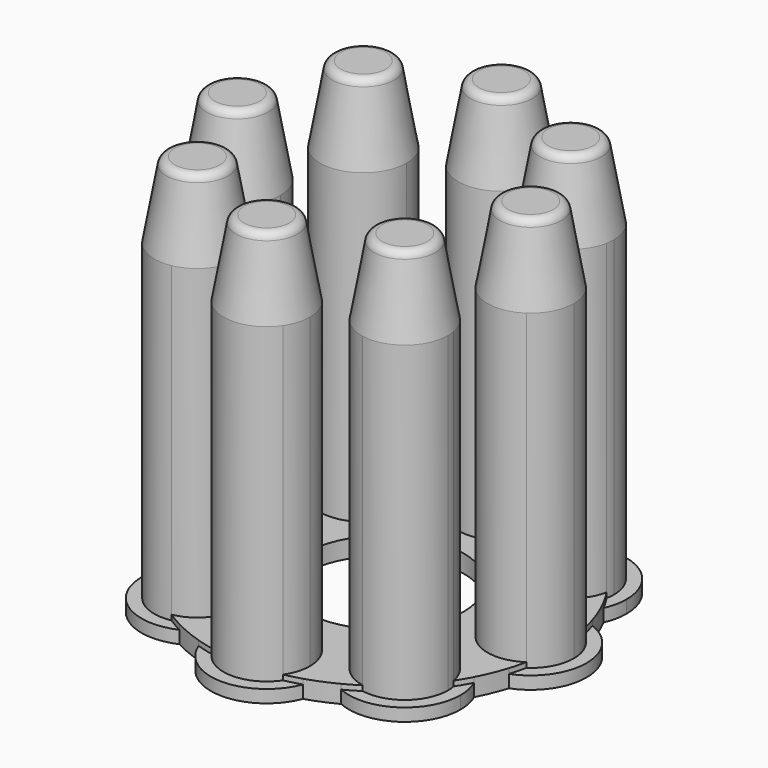
from build123d import *

# Parameters (mm, degrees)
F0_R            = 7.9375
F1_DEPTH        = 0.508
F2_DEPTH        = 1.27
F3_DEPTH        = 31.242
F5_COPIES_COUNT = 8


# Not quite as in the source:
# - a pattern or mirror of a feature is missing from the dataset's text; its kind, count and spacing are read off the source's solid


with BuildPart() as f1:
    # F0 (on Top) → F1 (new body)
    with BuildSketch(Plane.XY):
        with BuildLine():
            ThreePointArc((-5.219470135, 16.6642142857), (-1.0147277679, 9.1734047727), (5.588, 14.6685))
            ThreePointArc((5.588, 14.6685), (5.4950952273, 15.6832277679), (5.219470135, 16.6642142857))
            ThreePointArc((5.219470135, 16.6642142857), (4.4014869197, 16.8986928236), (3.573052384, 17.0930454545))
            ThreePointArc((3.573052384, 17.0930454545), (4.1275636999, 15.936704204), (4.318, 14.6685))
            ThreePointArc((4.318, 14.6685), (-1.268204204, 10.5409363001), (-3.573052384, 17.0930454545))
            ThreePointArc((-3.573052384, 17.0930454545), (-4.4014869197, 16.8986928236), (-5.219470135, 16.6642142857))
        make_face()
        with BuildLine():
            ThreePointArc((9.5600787818, 14.6131379223), (8.8368590405, 15.061501537), (8.0926561979, 15.4741016512))
            ThreePointArc((8.0926561979, 15.4741016512), (6.4208831266, 6.4208831266), (15.4741016512, 8.0926561979))
            ThreePointArc((15.4741016512, 8.0926561979), (15.061501537, 8.8368590405), (14.6131379223, 9.5600787818))
            ThreePointArc((14.6131379223, 9.5600787818), (7.3189087387, 7.3189087387), (9.5600787818, 14.6131379223))
        make_face()
        with BuildLine():
            ThreePointArc((17.0930454545, 3.573052384), (16.8986928236, 4.4014869197), (16.6642142857, 5.219470135))
            ThreePointArc((16.6642142857, 5.219470135), (9.0805, 0), (16.6642142857, -5.219470135))
            ThreePointArc((16.6642142857, -5.219470135), (16.8986928236, -4.4014869197), (17.0930454545, -3.573052384))
            ThreePointArc((17.0930454545, -3.573052384), (10.3505, 0), (17.0930454545, 3.573052384))
        make_face()
        with BuildLine():
            ThreePointArc((14.6131379223, -9.5600787818), (15.061501537, -8.8368590405), (15.4741016512, -8.0926561979))
            ThreePointArc((15.4741016512, -8.0926561979), (6.4208831266, -6.4208831266), (8.0926561979, -15.4741016512))
            ThreePointArc((8.0926561979, -15.4741016512), (8.8368590405, -15.061501537), (9.5600787818, -14.6131379223))
            ThreePointArc((9.5600787818, -14.6131379223), (7.3189087387, -7.3189087387), (14.6131379223, -9.5600787818))
        make_face()
        with BuildLine():
            ThreePointArc((3.573052384, -17.0930454545), (4.4014869197, -16.8986928236), (5.219470135, -16.6642142857))
            ThreePointArc((5.219470135, -16.6642142857), (5.4950952273, -15.6832277679), (5.588, -14.6685))
            ThreePointArc((5.588, -14.6685), (-1.0147277679, -9.1734047727), (-5.219470135, -16.6642142857))
            ThreePointArc((-5.219470135, -16.6642142857), (-4.4014869197, -16.8986928236), (-3.573052384, -17.0930454545))
            ThreePointArc((-3.573052384, -17.0930454545), (-1.268204204, -10.5409363001), (4.318, -14.6685))
            ThreePointArc((4.318, -14.6685), (4.1275636999, -15.936704204), (3.573052384, -17.0930454545))
        make_face()
        with BuildLine():
            ThreePointArc((-4.7841958198, -10.3721958198), (-9.2068001329, -4.907070305), (-15.4741016512, -8.0926561979))
            ThreePointArc((-15.4741016512, -8.0926561979), (-15.061501537, -8.8368590405), (-14.6131379223, -9.5600787818))
            ThreePointArc((-14.6131379223, -9.5600787818), (-9.9643134829, -6.0735034606), (-6.0541958198, -10.3721958198))
            ThreePointArc((-6.0541958198, -10.3721958198), (-7.044144936, -13.1234139709), (-9.5600787818, -14.6131379223))
            ThreePointArc((-9.5600787818, -14.6131379223), (-8.8368590405, -15.061501537), (-8.0926561979, -15.4741016512))
            ThreePointArc((-8.0926561979, -15.4741016512), (-5.6837093153, -13.4125639384), (-4.7841958198, -10.3721958198))
        make_face()
        with BuildLine():
            ThreePointArc((-9.0805, 0), (-11.5004017872, 4.6031399842), (-16.6642142857, 5.219470135))
            ThreePointArc((-16.6642142857, 5.219470135), (-16.8986928236, 4.4014869197), (-17.0930454545, 3.573052384))
            ThreePointArc((-17.0930454545, 3.573052384), (-12.6466275105, 3.8153840746), (-10.3505, 0))
            ThreePointArc((-10.3505, 0), (-12.6466275105, -3.8153840746), (-17.0930454545, -3.573052384))
            ThreePointArc((-17.0930454545, -3.573052384), (-16.8986928236, -4.4014869197), (-16.6642142857, -5.219470135))
            ThreePointArc((-16.6642142857, -5.219470135), (-11.5004017872, -4.6031399842), (-9.0805, 0))
        make_face()
        with BuildLine():
            ThreePointArc((-4.7841958198, 10.3721958198), (-5.6837093153, 13.4125639384), (-8.0926561979, 15.4741016512))
            ThreePointArc((-8.0926561979, 15.4741016512), (-8.8368590405, 15.061501537), (-9.5600787818, 14.6131379223))
            ThreePointArc((-9.5600787818, 14.6131379223), (-7.044144936, 13.1234139709), (-6.0541958198, 10.3721958198))
            ThreePointArc((-6.0541958198, 10.3721958198), (-9.9643134829, 6.0735034606), (-14.6131379223, 9.5600787818))
            ThreePointArc((-14.6131379223, 9.5600787818), (-15.061501537, 8.8368590405), (-15.4741016512, 8.0926561979))
            ThreePointArc((-15.4741016512, 8.0926561979), (-9.2068001329, 4.907070305), (-4.7841958198, 10.3721958198))
        make_face()
        with BuildLine():
            ThreePointArc((5.219470135, 16.6642142857), (5.4950952273, 15.6832277679), (5.588, 14.6685))
            ThreePointArc((5.588, 14.6685), (-1.0147277679, 9.1734047727), (-5.219470135, 16.6642142857))
            ThreePointArc((-5.219470135, 16.6642142857), (-6.6826094377, 16.1332463365), (-8.0926561979, 15.4741016512))
            ThreePointArc((-8.0926561979, 15.4741016512), (-5.6837093153, 13.4125639384), (-4.7841958198, 10.3721958198))
            ThreePointArc((-4.7841958198, 10.3721958198), (-9.2068001329, 4.907070305), (-15.4741016512, 8.0926561979))
            ThreePointArc((-15.4741016512, 8.0926561979), (-16.1332463365, 6.6826094377), (-16.6642142857, 5.219470135))
            ThreePointArc((-16.6642142857, 5.219470135), (-11.5004017872, 4.6031399842), (-9.0805, 0))
            ThreePointArc((-9.0805, 0), (-11.5004017872, -4.6031399842), (-16.6642142857, -5.219470135))
            ThreePointArc((-16.6642142857, -5.219470135), (-16.1332463365, -6.6826094377), (-15.4741016512, -8.0926561979))
            ThreePointArc((-15.4741016512, -8.0926561979), (-9.2068001329, -4.907070305), (-4.7841958198, -10.3721958198))
            ThreePointArc((-4.7841958198, -10.3721958198), (-5.6837093153, -13.4125639384), (-8.0926561979, -15.4741016512))
            ThreePointArc((-8.0926561979, -15.4741016512), (-6.6826094377, -16.1332463365), (-5.219470135, -16.6642142857))
            ThreePointArc((-5.219470135, -16.6642142857), (-1.0147277679, -9.1734047727), (5.588, -14.6685))
            ThreePointArc((5.588, -14.6685), (5.4950952273, -15.6832277679), (5.219470135, -16.6642142857))
            ThreePointArc((5.219470135, -16.6642142857), (6.6826094377, -16.1332463365), (8.0926561979, -15.4741016512))
            ThreePointArc((8.0926561979, -15.4741016512), (6.4208831266, -6.4208831266), (15.4741016512, -8.0926561979))
            ThreePointArc((15.4741016512, -8.0926561979), (16.1332463365, -6.6826094377), (16.6642142857, -5.219470135))
            ThreePointArc((16.6642142857, -5.219470135), (9.0805, 0), (16.6642142857, 5.219470135))
            ThreePointArc((16.6642142857, 5.219470135), (16.1332463365, 6.6826094377), (15.4741016512, 8.0926561979))
            ThreePointArc((15.4741016512, 8.0926561979), (6.4208831266, 6.4208831266), (8.0926561979, 15.4741016512))
            ThreePointArc((8.0926561979, 15.4741016512), (6.6826094377, 16.1332463365), (5.219470135, 16.6642142857))
        make_face()
        Circle(F0_R, mode=Mode.SUBTRACT)
    extrude(amount=F1_DEPTH)

    # F0 (on Top) → F2 (join)
    with BuildSketch(Plane.XY):
        with BuildLine():
            ThreePointArc((-5.219470135, 16.6642142857), (-1.0147277679, 9.1734047727), (5.588, 14.6685))
            ThreePointArc((5.588, 14.6685), (5.4950952273, 15.6832277679), (5.219470135, 16.6642142857))
            ThreePointArc((5.219470135, 16.6642142857), (4.4014869197, 16.8986928236), (3.573052384, 17.0930454545))
            ThreePointArc((3.573052384, 17.0930454545), (4.1275636999, 15.936704204), (4.318, 14.6685))
            ThreePointArc((4.318, 14.6685), (-1.268204204, 10.5409363001), (-3.573052384, 17.0930454545))
            ThreePointArc((-3.573052384, 17.0930454545), (-4.4014869197, 16.8986928236), (-5.219470135, 16.6642142857))
        make_face()
        with BuildLine():
            ThreePointArc((5.219470135, 16.6642142857), (5.4950952273, 15.6832277679), (5.588, 14.6685))
            ThreePointArc((5.588, 14.6685), (-1.0147277679, 9.1734047727), (-5.219470135, 16.6642142857))
            ThreePointArc((-5.219470135, 16.6642142857), (-6.6826094377, 16.1332463365), (-8.0926561979, 15.4741016512))
            ThreePointArc((-8.0926561979, 15.4741016512), (-5.6837093153, 13.4125639384), (-4.7841958198, 10.3721958198))
            ThreePointArc((-4.7841958198, 10.3721958198), (-9.2068001329, 4.907070305), (-15.4741016512, 8.0926561979))
            ThreePointArc((-15.4741016512, 8.0926561979), (-16.1332463365, 6.6826094377), (-16.6642142857, 5.219470135))
            ThreePointArc((-16.6642142857, 5.219470135), (-11.5004017872, 4.6031399842), (-9.0805, 0))
            ThreePointArc((-9.0805, 0), (-11.5004017872, -4.6031399842), (-16.6642142857, -5.219470135))
            ThreePointArc((-16.6642142857, -5.219470135), (-16.1332463365, -6.6826094377), (-15.4741016512, -8.0926561979))
            ThreePointArc((-15.4741016512, -8.0926561979), (-9.2068001329, -4.907070305), (-4.7841958198, -10.3721958198))
            ThreePointArc((-4.7841958198, -10.3721958198), (-5.6837093153, -13.4125639384), (-8.0926561979, -15.4741016512))
            ThreePointArc((-8.0926561979, -15.4741016512), (-6.6826094377, -16.1332463365), (-5.219470135, -16.6642142857))
            ThreePointArc((-5.219470135, -16.6642142857), (-1.0147277679, -9.1734047727), (5.588, -14.6685))
            ThreePointArc((5.588, -14.6685), (5.4950952273, -15.6832277679), (5.219470135, -16.6642142857))
            ThreePointArc((5.219470135, -16.6642142857), (6.6826094377, -16.1332463365), (8.0926561979, -15.4741016512))
            ThreePointArc((8.0926561979, -15.4741016512), (6.4208831266, -6.4208831266), (15.4741016512, -8.0926561979))
            ThreePointArc((15.4741016512, -8.0926561979), (16.1332463365, -6.6826094377), (16.6642142857, -5.219470135))
            ThreePointArc((16.6642142857, -5.219470135), (9.0805, 0), (16.6642142857, 5.219470135))
            ThreePointArc((16.6642142857, 5.219470135), (16.1332463365, 6.6826094377), (15.4741016512, 8.0926561979))
            ThreePointArc((15.4741016512, 8.0926561979), (6.4208831266, 6.4208831266), (8.0926561979, 15.4741016512))
            ThreePointArc((8.0926561979, 15.4741016512), (6.6826094377, 16.1332463365), (5.219470135, 16.6642142857))
        make_face()
        Circle(F0_R, mode=Mode.SUBTRACT)
        with BuildLine():
            ThreePointArc((3.573052384, 17.0930454545), (4.4014869197, 16.8986928236), (5.219470135, 16.6642142857))
            ThreePointArc((5.219470135, 16.6642142857), (0, 20.2565), (-5.219470135, 16.6642142857))
            ThreePointArc((-5.219470135, 16.6642142857), (-4.4014869197, 16.8986928236), (-3.573052384, 17.0930454545))
            ThreePointArc((-3.573052384, 17.0930454545), (0, 18.9865), (3.573052384, 17.0930454545))
        make_face()
        with BuildLine():
            ThreePointArc((15.9601958198, 10.3721958198), (13.4125639384, 15.0606823244), (8.0926561979, 15.4741016512))
            ThreePointArc((8.0926561979, 15.4741016512), (8.8368590405, 15.061501537), (9.5600787818, 14.6131379223))
            ThreePointArc((9.5600787818, 14.6131379223), (13.1234139709, 13.7002467036), (14.6901958198, 10.3721958198))
            ThreePointArc((14.6901958198, 10.3721958198), (14.6708881791, 9.9643134829), (14.6131379223, 9.5600787818))
            ThreePointArc((14.6131379223, 9.5600787818), (15.061501537, 8.8368590405), (15.4741016512, 8.0926561979))
            ThreePointArc((15.4741016512, 8.0926561979), (15.8373213347, 9.2068001329), (15.9601958198, 10.3721958198))
        make_face()
        with BuildLine():
            ThreePointArc((9.5600787818, 14.6131379223), (8.8368590405, 15.061501537), (8.0926561979, 15.4741016512))
            ThreePointArc((8.0926561979, 15.4741016512), (6.4208831266, 6.4208831266), (15.4741016512, 8.0926561979))
            ThreePointArc((15.4741016512, 8.0926561979), (15.061501537, 8.8368590405), (14.6131379223, 9.5600787818))
            ThreePointArc((14.6131379223, 9.5600787818), (7.3189087387, 7.3189087387), (9.5600787818, 14.6131379223))
        make_face()
        with BuildLine():
            ThreePointArc((-4.7841958198, 10.3721958198), (-5.6837093153, 13.4125639384), (-8.0926561979, 15.4741016512))
            ThreePointArc((-8.0926561979, 15.4741016512), (-8.8368590405, 15.061501537), (-9.5600787818, 14.6131379223))
            ThreePointArc((-9.5600787818, 14.6131379223), (-7.044144936, 13.1234139709), (-6.0541958198, 10.3721958198))
            ThreePointArc((-6.0541958198, 10.3721958198), (-9.9643134829, 6.0735034606), (-14.6131379223, 9.5600787818))
            ThreePointArc((-14.6131379223, 9.5600787818), (-15.061501537, 8.8368590405), (-15.4741016512, 8.0926561979))
            ThreePointArc((-15.4741016512, 8.0926561979), (-9.2068001329, 4.907070305), (-4.7841958198, 10.3721958198))
        make_face()
        with BuildLine():
            ThreePointArc((-9.5600787818, 14.6131379223), (-8.8368590405, 15.061501537), (-8.0926561979, 15.4741016512))
            ThreePointArc((-8.0926561979, 15.4741016512), (-14.3235085131, 14.3235085131), (-15.4741016512, 8.0926561979))
            ThreePointArc((-15.4741016512, 8.0926561979), (-15.061501537, 8.8368590405), (-14.6131379223, 9.5600787818))
            ThreePointArc((-14.6131379223, 9.5600787818), (-13.425482901, 13.425482901), (-9.5600787818, 14.6131379223))
        make_face()
        with BuildLine():
            ThreePointArc((20.2565, 0), (19.2716399842, 3.1680982128), (16.6642142857, 5.219470135))
            ThreePointArc((16.6642142857, 5.219470135), (16.8986928236, 4.4014869197), (17.0930454545, 3.573052384))
            ThreePointArc((17.0930454545, 3.573052384), (18.4838840746, 2.0218724895), (18.9865, 0))
            ThreePointArc((18.9865, 0), (18.4838840746, -2.0218724895), (17.0930454545, -3.573052384))
            ThreePointArc((17.0930454545, -3.573052384), (16.8986928236, -4.4014869197), (16.6642142857, -5.219470135))
            ThreePointArc((16.6642142857, -5.219470135), (19.2716399842, -3.1680982128), (20.2565, 0))
        make_face()
        with BuildLine():
            ThreePointArc((17.0930454545, 3.573052384), (16.8986928236, 4.4014869197), (16.6642142857, 5.219470135))
            ThreePointArc((16.6642142857, 5.219470135), (9.0805, 0), (16.6642142857, -5.219470135))
            ThreePointArc((16.6642142857, -5.219470135), (16.8986928236, -4.4014869197), (17.0930454545, -3.573052384))
            ThreePointArc((17.0930454545, -3.573052384), (10.3505, 0), (17.0930454545, 3.573052384))
        make_face()
        with BuildLine():
            ThreePointArc((-9.0805, 0), (-11.5004017872, 4.6031399842), (-16.6642142857, 5.219470135))
            ThreePointArc((-16.6642142857, 5.219470135), (-16.8986928236, 4.4014869197), (-17.0930454545, 3.573052384))
            ThreePointArc((-17.0930454545, 3.573052384), (-12.6466275105, 3.8153840746), (-10.3505, 0))
            ThreePointArc((-10.3505, 0), (-12.6466275105, -3.8153840746), (-17.0930454545, -3.573052384))
            ThreePointArc((-17.0930454545, -3.573052384), (-16.8986928236, -4.4014869197), (-16.6642142857, -5.219470135))
            ThreePointArc((-16.6642142857, -5.219470135), (-11.5004017872, -4.6031399842), (-9.0805, 0))
        make_face()
        with BuildLine():
            ThreePointArc((-17.0930454545, 3.573052384), (-16.8986928236, 4.4014869197), (-16.6642142857, 5.219470135))
            ThreePointArc((-16.6642142857, 5.219470135), (-20.2565, 0), (-16.6642142857, -5.219470135))
            ThreePointArc((-16.6642142857, -5.219470135), (-16.8986928236, -4.4014869197), (-17.0930454545, -3.573052384))
            ThreePointArc((-17.0930454545, -3.573052384), (-18.9865, 0), (-17.0930454545, 3.573052384))
        make_face()
        with BuildLine():
            ThreePointArc((15.9601958198, -10.3721958198), (15.8373213347, -9.2068001329), (15.4741016512, -8.0926561979))
            ThreePointArc((15.4741016512, -8.0926561979), (15.061501537, -8.8368590405), (14.6131379223, -9.5600787818))
            ThreePointArc((14.6131379223, -9.5600787818), (14.6708881791, -9.9643134829), (14.6901958198, -10.3721958198))
            ThreePointArc((14.6901958198, -10.3721958198), (13.1234139709, -13.7002467036), (9.5600787818, -14.6131379223))
            ThreePointArc((9.5600787818, -14.6131379223), (8.8368590405, -15.061501537), (8.0926561979, -15.4741016512))
            ThreePointArc((8.0926561979, -15.4741016512), (13.4125639384, -15.0606823244), (15.9601958198, -10.3721958198))
        make_face()
        with BuildLine():
            ThreePointArc((14.6131379223, -9.5600787818), (15.061501537, -8.8368590405), (15.4741016512, -8.0926561979))
            ThreePointArc((15.4741016512, -8.0926561979), (6.4208831266, -6.4208831266), (8.0926561979, -15.4741016512))
            ThreePointArc((8.0926561979, -15.4741016512), (8.8368590405, -15.061501537), (9.5600787818, -14.6131379223))
            ThreePointArc((9.5600787818, -14.6131379223), (7.3189087387, -7.3189087387), (14.6131379223, -9.5600787818))
        make_face()
        with BuildLine():
            ThreePointArc((-4.7841958198, -10.3721958198), (-9.2068001329, -4.907070305), (-15.4741016512, -8.0926561979))
            ThreePointArc((-15.4741016512, -8.0926561979), (-15.061501537, -8.8368590405), (-14.6131379223, -9.5600787818))
            ThreePointArc((-14.6131379223, -9.5600787818), (-9.9643134829, -6.0735034606), (-6.0541958198, -10.3721958198))
            ThreePointArc((-6.0541958198, -10.3721958198), (-7.044144936, -13.1234139709), (-9.5600787818, -14.6131379223))
            ThreePointArc((-9.5600787818, -14.6131379223), (-8.8368590405, -15.061501537), (-8.0926561979, -15.4741016512))
            ThreePointArc((-8.0926561979, -15.4741016512), (-5.6837093153, -13.4125639384), (-4.7841958198, -10.3721958198))
        make_face()
        with BuildLine():
            ThreePointArc((-14.6131379223, -9.5600787818), (-15.061501537, -8.8368590405), (-15.4741016512, -8.0926561979))
            ThreePointArc((-15.4741016512, -8.0926561979), (-14.3235085131, -14.3235085131), (-8.0926561979, -15.4741016512))
            ThreePointArc((-8.0926561979, -15.4741016512), (-8.8368590405, -15.061501537), (-9.5600787818, -14.6131379223))
            ThreePointArc((-9.5600787818, -14.6131379223), (-13.425482901, -13.425482901), (-14.6131379223, -9.5600787818))
        make_face()
        with BuildLine():
            ThreePointArc((-5.219470135, -16.6642142857), (0, -20.2565), (5.219470135, -16.6642142857))
            ThreePointArc((5.219470135, -16.6642142857), (4.4014869197, -16.8986928236), (3.573052384, -17.0930454545))
            ThreePointArc((3.573052384, -17.0930454545), (0, -18.9865), (-3.573052384, -17.0930454545))
            ThreePointArc((-3.573052384, -17.0930454545), (-4.4014869197, -16.8986928236), (-5.219470135, -16.6642142857))
        make_face()
        with BuildLine():
            ThreePointArc((3.573052384, -17.0930454545), (4.4014869197, -16.8986928236), (5.219470135, -16.6642142857))
            ThreePointArc((5.219470135, -16.6642142857), (5.4950952273, -15.6832277679), (5.588, -14.6685))
            ThreePointArc((5.588, -14.6685), (-1.0147277679, -9.1734047727), (-5.219470135, -16.6642142857))
            ThreePointArc((-5.219470135, -16.6642142857), (-4.4014869197, -16.8986928236), (-3.573052384, -17.0930454545))
            ThreePointArc((-3.573052384, -17.0930454545), (-1.268204204, -10.5409363001), (4.318, -14.6685))
            ThreePointArc((4.318, -14.6685), (4.1275636999, -15.936704204), (3.573052384, -17.0930454545))
        make_face()
        with BuildLine():
            ThreePointArc((-3.573052384, -17.0930454545), (0, -18.9865), (3.573052384, -17.0930454545))
            ThreePointArc((3.573052384, -17.0930454545), (0, -17.4625), (-3.573052384, -17.0930454545))
        make_face()
        with BuildLine():
            ThreePointArc((-3.573052384, -17.0930454545), (0, -17.4625), (3.573052384, -17.0930454545))
            ThreePointArc((3.573052384, -17.0930454545), (4.1275636999, -15.936704204), (4.318, -14.6685))
            ThreePointArc((4.318, -14.6685), (-1.268204204, -10.5409363001), (-3.573052384, -17.0930454545))
        make_face()
        with BuildLine():
            ThreePointArc((9.5600787818, -14.6131379223), (12.3478521665, -12.3478521665), (14.6131379223, -9.5600787818))
            ThreePointArc((14.6131379223, -9.5600787818), (7.3189087387, -7.3189087387), (9.5600787818, -14.6131379223))
        make_face()
        with BuildLine():
            ThreePointArc((14.6901958198, -10.3721958198), (14.6708881791, -9.9643134829), (14.6131379223, -9.5600787818))
            ThreePointArc((14.6131379223, -9.5600787818), (12.3478521665, -12.3478521665), (9.5600787818, -14.6131379223))
            ThreePointArc((9.5600787818, -14.6131379223), (13.1234139709, -13.7002467036), (14.6901958198, -10.3721958198))
        make_face()
        with BuildLine():
            ThreePointArc((18.9865, 0), (18.4838840746, 2.0218724895), (17.0930454545, 3.573052384))
            ThreePointArc((17.0930454545, 3.573052384), (17.3698907956, 1.7960512242), (17.4625, 0))
            ThreePointArc((17.4625, 0), (17.3698907956, -1.7960512242), (17.0930454545, -3.573052384))
            ThreePointArc((17.0930454545, -3.573052384), (18.4838840746, -2.0218724895), (18.9865, 0))
        make_face()
        with BuildLine():
            ThreePointArc((17.4625, 0), (17.3698907956, 1.7960512242), (17.0930454545, 3.573052384))
            ThreePointArc((17.0930454545, 3.573052384), (10.3505, 0), (17.0930454545, -3.573052384))
            ThreePointArc((17.0930454545, -3.573052384), (17.3698907956, -1.7960512242), (17.4625, 0))
        make_face()
        with BuildLine():
            ThreePointArc((14.6131379223, 9.5600787818), (12.3478521665, 12.3478521665), (9.5600787818, 14.6131379223))
            ThreePointArc((9.5600787818, 14.6131379223), (7.3189087387, 7.3189087387), (14.6131379223, 9.5600787818))
        make_face()
        with BuildLine():
            ThreePointArc((14.6901958198, 10.3721958198), (13.1234139709, 13.7002467036), (9.5600787818, 14.6131379223))
            ThreePointArc((9.5600787818, 14.6131379223), (12.3478521665, 12.3478521665), (14.6131379223, 9.5600787818))
            ThreePointArc((14.6131379223, 9.5600787818), (14.6708881791, 9.9643134829), (14.6901958198, 10.3721958198))
        make_face()
        with BuildLine():
            ThreePointArc((-6.0541958198, 10.3721958198), (-7.044144936, 13.1234139709), (-9.5600787818, 14.6131379223))
            ThreePointArc((-9.5600787818, 14.6131379223), (-12.3478521665, 12.3478521665), (-14.6131379223, 9.5600787818))
            ThreePointArc((-14.6131379223, 9.5600787818), (-9.9643134829, 6.0735034606), (-6.0541958198, 10.3721958198))
        make_face()
        with BuildLine():
            ThreePointArc((-14.6131379223, 9.5600787818), (-12.3478521665, 12.3478521665), (-9.5600787818, 14.6131379223))
            ThreePointArc((-9.5600787818, 14.6131379223), (-13.425482901, 13.425482901), (-14.6131379223, 9.5600787818))
        make_face()
        with BuildLine():
            ThreePointArc((-10.3505, 0), (-12.6466275105, 3.8153840746), (-17.0930454545, 3.573052384))
            ThreePointArc((-17.0930454545, 3.573052384), (-17.4625, 0), (-17.0930454545, -3.573052384))
            ThreePointArc((-17.0930454545, -3.573052384), (-12.6466275105, -3.8153840746), (-10.3505, 0))
        make_face()
        with BuildLine():
            ThreePointArc((4.318, 14.6685), (4.1275636999, 15.936704204), (3.573052384, 17.0930454545))
            ThreePointArc((3.573052384, 17.0930454545), (0, 17.4625), (-3.573052384, 17.0930454545))
            ThreePointArc((-3.573052384, 17.0930454545), (-1.268204204, 10.5409363001), (4.318, 14.6685))
        make_face()
        with BuildLine():
            ThreePointArc((-3.573052384, 17.0930454545), (0, 17.4625), (3.573052384, 17.0930454545))
            ThreePointArc((3.573052384, 17.0930454545), (0, 18.9865), (-3.573052384, 17.0930454545))
        make_face()
        with BuildLine():
            ThreePointArc((-9.5600787818, -14.6131379223), (-12.3478521665, -12.3478521665), (-14.6131379223, -9.5600787818))
            ThreePointArc((-14.6131379223, -9.5600787818), (-13.425482901, -13.425482901), (-9.5600787818, -14.6131379223))
        make_face()
        with BuildLine():
            ThreePointArc((-6.0541958198, -10.3721958198), (-9.9643134829, -6.0735034606), (-14.6131379223, -9.5600787818))
            ThreePointArc((-14.6131379223, -9.5600787818), (-12.3478521665, -12.3478521665), (-9.5600787818, -14.6131379223))
            ThreePointArc((-9.5600787818, -14.6131379223), (-7.044144936, -13.1234139709), (-6.0541958198, -10.3721958198))
        make_face()
        with BuildLine():
            ThreePointArc((-17.0930454545, -3.573052384), (-17.4625, 0), (-17.0930454545, 3.573052384))
            ThreePointArc((-17.0930454545, 3.573052384), (-18.9865, 0), (-17.0930454545, -3.573052384))
        make_face()
    extrude(amount=-F2_DEPTH)

    # F0 (on Top) → F3 (join)
    with BuildSketch(Plane.XY):
        with BuildLine():
            ThreePointArc((9.5600787818, -14.6131379223), (12.3478521665, -12.3478521665), (14.6131379223, -9.5600787818))
            ThreePointArc((14.6131379223, -9.5600787818), (7.3189087387, -7.3189087387), (9.5600787818, -14.6131379223))
        make_face()
        with BuildLine():
            ThreePointArc((14.6901958198, -10.3721958198), (14.6708881791, -9.9643134829), (14.6131379223, -9.5600787818))
            ThreePointArc((14.6131379223, -9.5600787818), (12.3478521665, -12.3478521665), (9.5600787818, -14.6131379223))
            ThreePointArc((9.5600787818, -14.6131379223), (13.1234139709, -13.7002467036), (14.6901958198, -10.3721958198))
        make_face()
        with BuildLine():
            ThreePointArc((-3.573052384, -17.0930454545), (0, -18.9865), (3.573052384, -17.0930454545))
            ThreePointArc((3.573052384, -17.0930454545), (0, -17.4625), (-3.573052384, -17.0930454545))
        make_face()
        with BuildLine():
            ThreePointArc((-3.573052384, -17.0930454545), (0, -17.4625), (3.573052384, -17.0930454545))
            ThreePointArc((3.573052384, -17.0930454545), (4.1275636999, -15.936704204), (4.318, -14.6685))
            ThreePointArc((4.318, -14.6685), (-1.268204204, -10.5409363001), (-3.573052384, -17.0930454545))
        make_face()
        with BuildLine():
            ThreePointArc((-6.0541958198, -10.3721958198), (-9.9643134829, -6.0735034606), (-14.6131379223, -9.5600787818))
            ThreePointArc((-14.6131379223, -9.5600787818), (-12.3478521665, -12.3478521665), (-9.5600787818, -14.6131379223))
            ThreePointArc((-9.5600787818, -14.6131379223), (-7.044144936, -13.1234139709), (-6.0541958198, -10.3721958198))
        make_face()
        with BuildLine():
            ThreePointArc((-9.5600787818, -14.6131379223), (-12.3478521665, -12.3478521665), (-14.6131379223, -9.5600787818))
            ThreePointArc((-14.6131379223, -9.5600787818), (-13.425482901, -13.425482901), (-9.5600787818, -14.6131379223))
        make_face()
        with BuildLine():
            ThreePointArc((-10.3505, 0), (-12.6466275105, 3.8153840746), (-17.0930454545, 3.573052384))
            ThreePointArc((-17.0930454545, 3.573052384), (-17.4625, 0), (-17.0930454545, -3.573052384))
            ThreePointArc((-17.0930454545, -3.573052384), (-12.6466275105, -3.8153840746), (-10.3505, 0))
        make_face()
        with BuildLine():
            ThreePointArc((-17.0930454545, -3.573052384), (-17.4625, 0), (-17.0930454545, 3.573052384))
            ThreePointArc((-17.0930454545, 3.573052384), (-18.9865, 0), (-17.0930454545, -3.573052384))
        make_face()
        with BuildLine():
            ThreePointArc((-6.0541958198, 10.3721958198), (-7.044144936, 13.1234139709), (-9.5600787818, 14.6131379223))
            ThreePointArc((-9.5600787818, 14.6131379223), (-12.3478521665, 12.3478521665), (-14.6131379223, 9.5600787818))
            ThreePointArc((-14.6131379223, 9.5600787818), (-9.9643134829, 6.0735034606), (-6.0541958198, 10.3721958198))
        make_face()
        with BuildLine():
            ThreePointArc((-14.6131379223, 9.5600787818), (-12.3478521665, 12.3478521665), (-9.5600787818, 14.6131379223))
            ThreePointArc((-9.5600787818, 14.6131379223), (-13.425482901, 13.425482901), (-14.6131379223, 9.5600787818))
        make_face()
        with BuildLine():
            ThreePointArc((4.318, 14.6685), (4.1275636999, 15.936704204), (3.573052384, 17.0930454545))
            ThreePointArc((3.573052384, 17.0930454545), (0, 17.4625), (-3.573052384, 17.0930454545))
            ThreePointArc((-3.573052384, 17.0930454545), (-1.268204204, 10.5409363001), (4.318, 14.6685))
        make_face()
        with BuildLine():
            ThreePointArc((-3.573052384, 17.0930454545), (0, 17.4625), (3.573052384, 17.0930454545))
            ThreePointArc((3.573052384, 17.0930454545), (0, 18.9865), (-3.573052384, 17.0930454545))
        make_face()
        with BuildLine():
            ThreePointArc((14.6131379223, 9.5600787818), (12.3478521665, 12.3478521665), (9.5600787818, 14.6131379223))
            ThreePointArc((9.5600787818, 14.6131379223), (7.3189087387, 7.3189087387), (14.6131379223, 9.5600787818))
        make_face()
        with BuildLine():
            ThreePointArc((14.6901958198, 10.3721958198), (13.1234139709, 13.7002467036), (9.5600787818, 14.6131379223))
            ThreePointArc((9.5600787818, 14.6131379223), (12.3478521665, 12.3478521665), (14.6131379223, 9.5600787818))
            ThreePointArc((14.6131379223, 9.5600787818), (14.6708881791, 9.9643134829), (14.6901958198, 10.3721958198))
        make_face()
        with BuildLine():
            ThreePointArc((17.4625, 0), (17.3698907956, 1.7960512242), (17.0930454545, 3.573052384))
            ThreePointArc((17.0930454545, 3.573052384), (10.3505, 0), (17.0930454545, -3.573052384))
            ThreePointArc((17.0930454545, -3.573052384), (17.3698907956, -1.7960512242), (17.4625, 0))
        make_face()
        with BuildLine():
            ThreePointArc((18.9865, 0), (18.4838840746, 2.0218724895), (17.0930454545, 3.573052384))
            ThreePointArc((17.0930454545, 3.573052384), (17.3698907956, 1.7960512242), (17.4625, 0))
            ThreePointArc((17.4625, 0), (17.3698907956, -1.7960512242), (17.0930454545, -3.573052384))
            ThreePointArc((17.0930454545, -3.573052384), (18.4838840746, -2.0218724895), (18.9865, 0))
        make_face()
    extrude(amount=F3_DEPTH)

    # F4 (on Right) → F5 (revolve)
    with BuildSketch(Plane.YZ):
        with BuildLine():
            Line((14.6685, 38.862), (14.6685, 31.242))
            Line((14.6685, 31.242), (18.9865, 31.242))
            Line((18.9865, 31.242), (17.7662546168, 38.1623554571))
            ThreePointArc((17.7662546168, 38.1623554571), (17.4766775621, 38.6639176285), (16.9324507193, 38.862))
            Line((16.9324507193, 38.862), (14.6685, 38.862))
        make_face()
    f5 = revolve(axis=Axis((0, 14.6685, 35.052), (0, 0, 1)))

    # F5_copies: F5 ×8 about axis
    f5_copies_axis = Axis((0, 0, 0), (0, 0, 1))
    for i in range(1, F5_COPIES_COUNT):
        add(f5.rotate(f5_copies_axis, i * 360 / F5_COPIES_COUNT))


solid = f1.part
